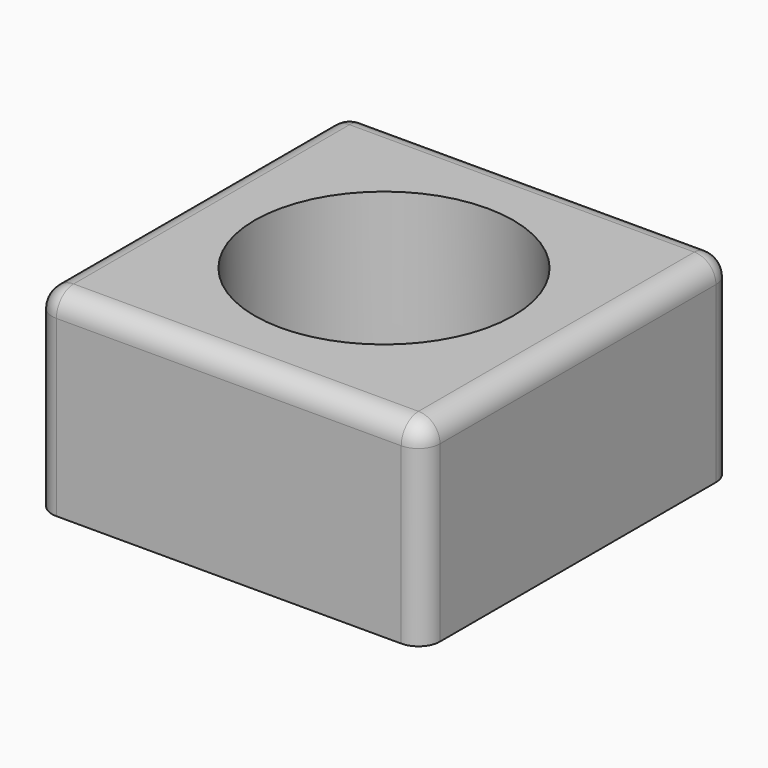
from build123d import *

# Parameters (mm, degrees)
F0_W        = 90
F0_H        = 90
F1_DEPTH    = 45.4
F2_R        = 30
F3_DEPTH    = 45.401
F4_R        = 5
F5_T1_DEPTH = 52.9
F5_S5_W     = 5
F5_S5_H     = 5
F5_T6_DEPTH = 5


# Not quite as in the source:
# - a fillet or chamfer that OpenCascade refuses, or shapes differently, is made with other operations: its cross-section is extruded or revolved along the edge and cut away or added


with BuildPart() as f1:
    # F0 (on Top) → F1 (new body)
    with BuildSketch(Plane.XY):
        Rectangle(F0_W, F0_H)
    extrude(amount=F1_DEPTH)

    # F2 (on face) → F3 (cut, through all)
    with BuildSketch(Plane.XY.offset(45.4)):
        Circle(F2_R)
    extrude(amount=-F3_DEPTH, mode=Mode.SUBTRACT)

    # F4
    f4_edges = [f1.edges().sort_by_distance(p)[0] for p in [
        (-45, 45, 22.7),
        (-45, -45, 22.7),
        (45, 45, 22.7),
        (45, 0, 45.4),
        (-45, 0, 45.4),
        (0, 45, 45.4),
        (0, -45, 45.4),
    ]]
    fillet(f4_edges, radius=F4_R)

    # F5: fillet of radius 5 on 1 edges, made by hand

    # F5_s2 → F5_t1 (cut)
    with BuildSketch(Plane.XY.offset(-12.5)):
        with BuildLine():
            ThreePointArc((45, -40), (43.5355339059, -43.5355339059), (40, -45))
            Line((40, -45), (45, -45))
            Line((45, -45), (45, -40))
        make_face()
    extrude(amount=F5_T1_DEPTH, mode=Mode.SUBTRACT)


with BuildPart() as f5_tool4:
    # F5_s5 → F5_t6 (new body)
    with BuildSketch(Plane.YZ.offset(40)):
        with Locations((-42.5, 42.9)):
            Rectangle(F5_S5_W, F5_S5_H)
    extrude(amount=F5_T6_DEPTH)

    # F5_s7 → F5_t8 (revolve, cut)
    with BuildSketch(Plane(origin=(40, -40, 40.4), x_dir=(0, 0.7071067812, -0.7071067812), z_dir=(0, -0.7071067812, -0.7071067812))):
        with BuildLine():
            ThreePointArc((0, -5), (5, 0), (0, 5))
            Line((0, 5), (0, -5))
        make_face()
    revolve(axis=Axis((40, -40, 40.4), (1, 0, 0)), mode=Mode.SUBTRACT)


with BuildPart() as f1_1:
    add(f1.part)

    # F5_t3: cut F5_tool4
    add(f5_tool4.part, mode=Mode.SUBTRACT)


solid = f1_1.part
